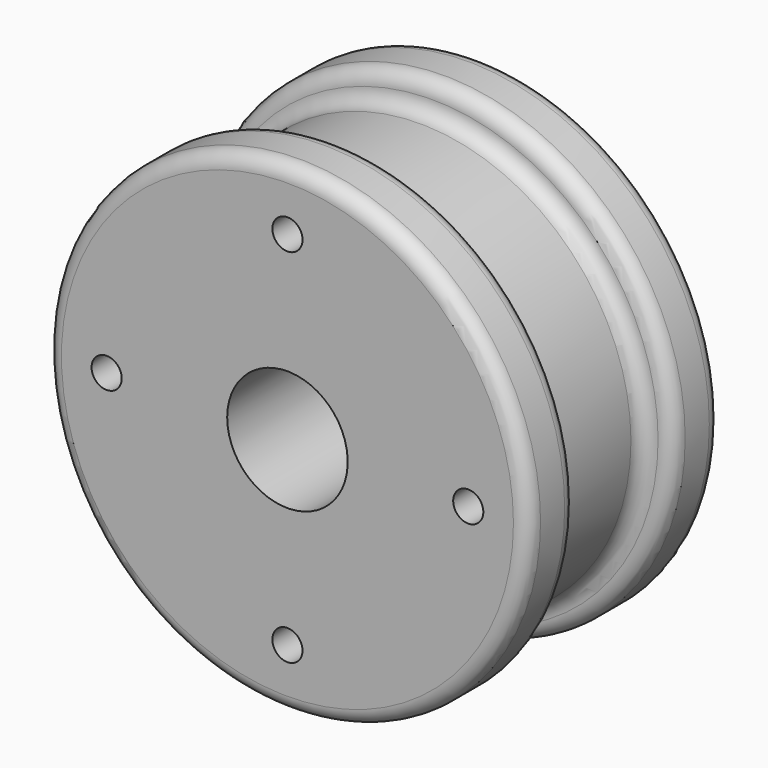
from build123d import *

# Parameters (mm, degrees)
F0_R     = 25.4
F1_DEPTH = 6.35
F2_R     = 22.225
F3_DEPTH = 12.7
F4_R     = 25.4
F5_DEPTH = 6.35
F7_D     = 3.175
F7_DEPTH = 3.175
F7_TIP   = 0.9538662327
F8_D     = 12.7
F9_R     = 1.58749


# Not quite as in the source:
# - a fillet or chamfer is up to 0.001 mm smaller than in the source, because OpenCascade refuses the exact size


with BuildPart() as f1:
    # F0 (on Front) → F1 (new body)
    with BuildSketch(Plane.XZ):
        Circle(F0_R)
    extrude(amount=F1_DEPTH)

    # F2 (on face) → F3 (join)
    with BuildSketch(Plane.XZ.offset(6.35)):
        Circle(F2_R)
    extrude(amount=F3_DEPTH)

    # F4 (on face) → F5 (join)
    with BuildSketch(Plane.XZ.offset(19.05)):
        Circle(F4_R)
    extrude(amount=F5_DEPTH)

    # F7
    with Locations(Plane.XZ.offset(25.4)):
        with Locations((0, 19.05), (-19.05, 0), (0, -19.05), (19.05, 0)):
            Hole(F7_D / 2, depth=F7_DEPTH)
            with Locations((0, 0, -(F7_DEPTH + F7_TIP / 2))):  # 118° drill point
                Cone(0, F7_D / 2, F7_TIP, mode=Mode.SUBTRACT)

    # F8 (through all)
    with Locations(Plane.XZ.offset(25.4)):
        with Locations((0, 0)):
            Hole(F8_D / 2)

    # F9 (radius 1.5875 in the source; OpenCascade refuses exactly that, so slightly less here)
    f9_edges = [f1.edges().sort_by_distance(p)[0] for p in [
        (-25.4, -25.4, 0),
        (-25.4, -6.35, 0),
        (-25.4, 0, 0),
        (-25.4, -19.05, 0),
        (-22.225, -6.35, 0),
        (-22.225, -19.05, 0),
    ]]
    fillet(f9_edges, radius=F9_R)


solid = f1.part
